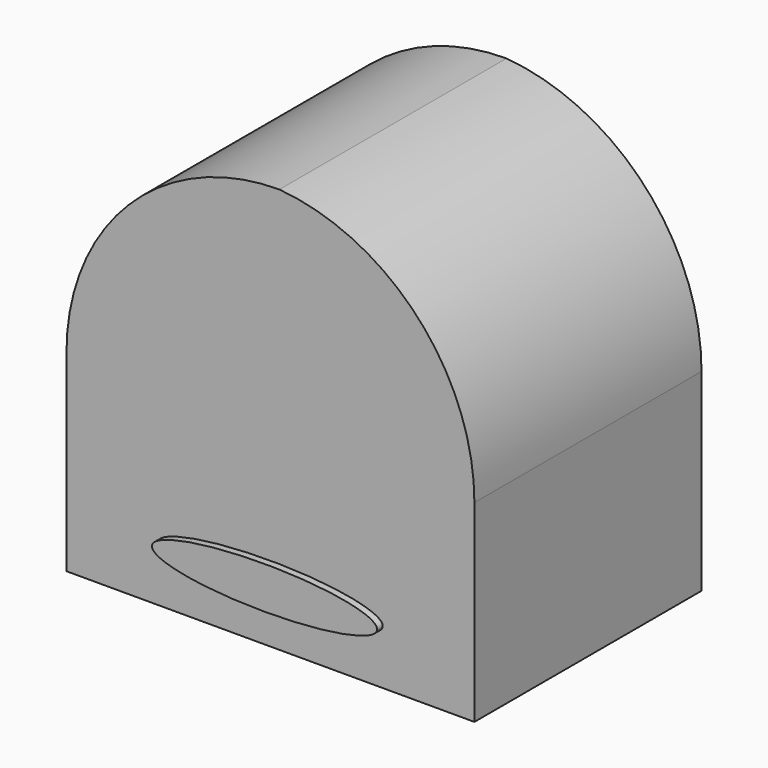
from build123d import *

# Parameters (mm, degrees)
F0_W        = 145.98980546
F0_H        = 145.0418308377
F1_DEPTH    = 101.6
F2_R        = 76.2
F3_T1_DEPTH = 481.2494898574
F5_DEPTH    = 2.54


# Not quite as in the source:
# - a fillet or chamfer that OpenCascade refuses, or shapes differently, is made with other operations: its cross-section is extruded or revolved along the edge and cut away or added


with BuildPart() as f1:
    # F0 (on Front) → F1 (new body)
    with BuildSketch(Plane.XZ):
        with Locations((0.0947937369, 0.9479857981)):
            Rectangle(F0_W, F0_H)
    extrude(amount=F1_DEPTH)

    # F2
    f2_edges = [f1.edges().sort_by_distance(p)[0] for p in [
        (-72.900109, -50.8, 73.468901),
    ]]
    fillet(f2_edges, radius=F2_R)

    # F3: fillet of radius 76.2 on 1 edges, made by hand

    # F3_s2 → F3_t1 (cut)
    with BuildSketch(Plane.XZ.offset(-189.8247449287)):
        with BuildLine():
            ThreePointArc((3.2998910069, 73.468901217), (52.9918213106, 49.1044140169), (73.0896964669, -2.4609967545))
            Line((73.0896964669, -2.4609967545), (73.0896964669, 73.468901217))
            Line((73.0896964669, 73.468901217), (3.2998910069, 73.468901217))
        make_face()
    extrude(amount=F3_T1_DEPTH, mode=Mode.SUBTRACT)

    # F4 (on face) → F5 (join)
    with BuildSketch(Plane.XZ.offset(101.6)):
        with BuildLine():
            add(Edge.make_bspline(
                [(40.2893982828, -52.0444214344), (40.2893982828, -38.976719833), (-20.1446991414, -45.5105706337), (-80.5787965655, -52.0444214344), (-20.1446991414, -58.5782722351), (40.2893982828, -65.1121230358), (40.2893982828, -52.0444214344)],
                knots=[0, 0, 0, 2.0943951024, 2.0943951024, 4.1887902048, 4.1887902048, 6.2831853072, 6.2831853072, 6.2831853072], degree=2, weights=[1, 0.5, 1, 0.5, 1, 0.5, 1]))
        make_face()
    extrude(amount=F5_DEPTH)


solid = f1.part
